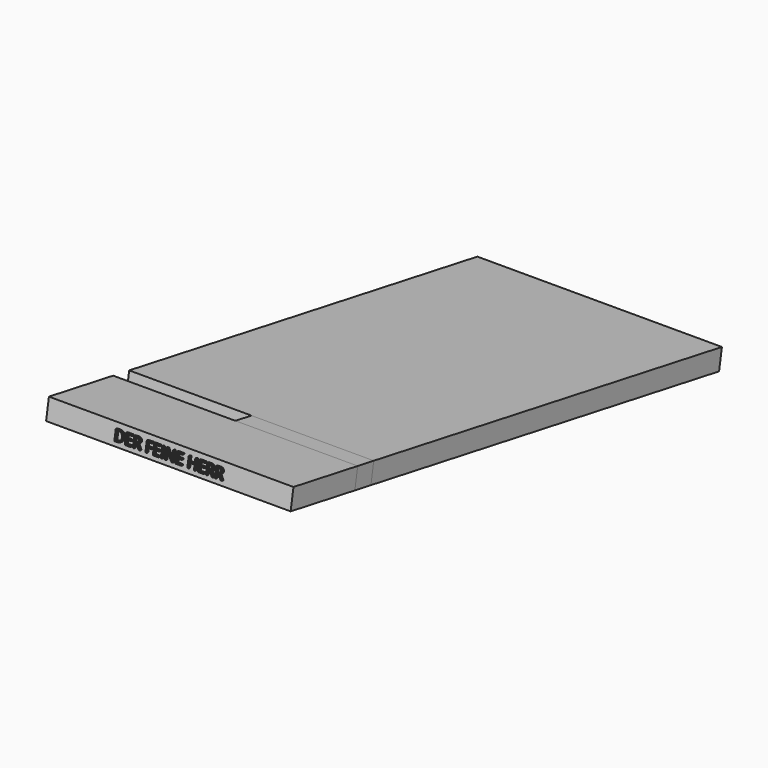
from build123d import *

# Parameters (mm, degrees)
F1_DEPTH     = 60
F2_DEPTH     = 60
F3_TEXT_SIZE = 7.0415954623
F4_DEPTH     = 1


# Not quite as in the source:
# - Text() gives the source's letters only with a copy of the font that has no kerning and outlines rounded to 1/6400 em; it was checked with that copy


with BuildPart() as f1:
    # F0 (on Right) → F1 (new body, symmetric)
    with BuildSketch(Plane.YZ):
        Polygon((-32.4463830138, -70.7629137145), (6.9459271067, -77.7088408211), (8.6824088833, -67.860763291), (-30.7099012371, -60.9148361843), align=None)
    extrude(amount=F1_DEPTH, both=True)

    # F3 (on face) → F4 (join)
    with BuildSketch(Plane(origin=(0, -19.3668339062, 3.4148953486), x_dir=(1, 0, 0), z_dir=(0, -0.984807753, 0.1736481777))):
        with Locations((-26.7476103885, -72.8570967913)):
            Text('DER FEINE HERR', F3_TEXT_SIZE, font='Open Sans', text_align=(TextAlign.LEFT, TextAlign.BOTTOM))
    extrude(amount=F4_DEPTH)


with BuildPart() as f1b:
    # F0 (on Right) → F1, piece 2 (new body, symmetric)
    with BuildSketch(Plane.YZ):
        Polygon((18.5304864135, -69.5972450677), (16.7940046368, -79.4453225978), (230.3508193257, -117.1011509416), (232.0873011024, -107.2530734115), align=None)
    extrude(amount=F1_DEPTH, both=True)


with BuildPart() as f2:
    # F0 (on Right) → F2 (new body)
    with BuildSketch(Plane.YZ):
        Polygon((8.6824088833, -67.860763291), (6.9459271067, -77.7088408211), (16.7940046368, -79.4453225978), (18.5304864135, -69.5972450677), align=None)
    extrude(amount=F2_DEPTH)


solid = Compound([f1.part, f1b.part, f2.part])
